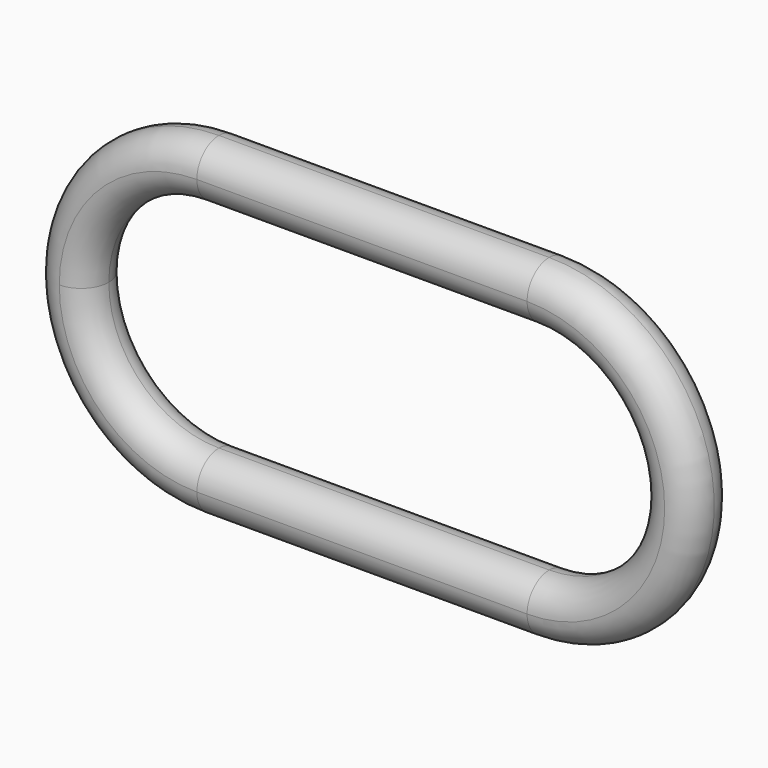
from build123d import *

# Parameters (mm, degrees)
F1_DEPTH      = 2.5
F1_DEPTH_BACK = 2.5
F2_R          = 2.49999


# Not quite as in the source:
# - a fillet or chamfer is up to 0.001 mm smaller than in the source, because OpenCascade refuses the exact size


with BuildPart() as f1:
    # F0 (on Front) → F1 (new body, two sides)
    with BuildSketch(Plane.XZ) as f1_sk:
        with BuildLine():
            ThreePointArc((15, -15), (25.6066017178, -10.6066017178), (30, 0))
            ThreePointArc((30, 0), (25.6066017178, 10.6066017178), (15, 15))
            Line((15, 15), (-15, 15))
            ThreePointArc((-15, 15), (-25.6066017178, 10.6066017178), (-30, 0))
            ThreePointArc((-30, 0), (-25.6066017178, -10.6066017178), (-15, -15))
            Line((-15, -15), (15, -15))
        make_face()
        with BuildLine():
            ThreePointArc((25, 0), (22.0710678119, -7.0710678119), (15, -10))
            Line((15, -10), (-15, -10))
            ThreePointArc((-15, -10), (-22.0710678119, -7.0710678119), (-25, 0))
            ThreePointArc((-25, 0), (-22.0710678119, 7.0710678119), (-15, 10))
            Line((-15, 10), (15, 10))
            ThreePointArc((15, 10), (22.0710678119, 7.0710678119), (25, 0))
        make_face(mode=Mode.SUBTRACT)
    extrude(amount=F1_DEPTH)
    extrude(f1_sk.sketch, amount=-F1_DEPTH_BACK)

    # F2 (radius 2.5 in the source; OpenCascade refuses exactly that, so slightly less here)
    f2_edges = [f1.edges().sort_by_distance(p)[0] for p in [
        (0, -2.5, -15),
        (0, 2.5, -15),
        (0, -2.5, -10),
        (0, 2.5, -10),
    ]]
    fillet(f2_edges, radius=F2_R)


solid = f1.part
